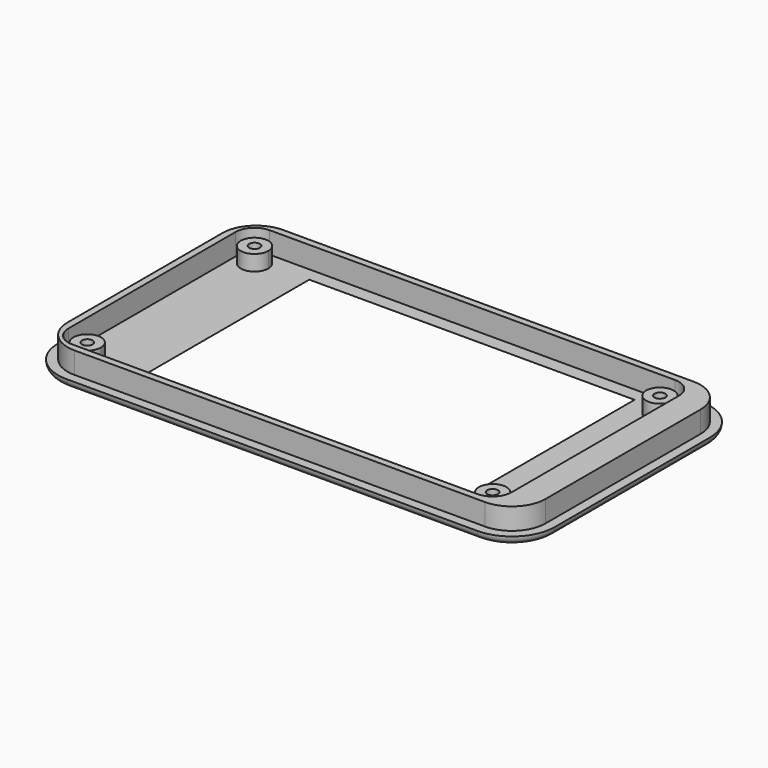
from build123d import *

# Parameters (mm, degrees)
F1_DEPTH = 5.6
F2_DEPTH = 7
F0_W     = 75.5
F0_H     = 51
F3_DEPTH = 2
F4_R     = 1.99999
F5_SIZE2 = 1.99999
F5_SIZE  = 2.99999
F6_R     = 1.25
F7_DEPTH = 5


# Not quite as in the source:
# - a fillet or chamfer is up to 0.001 mm smaller than in the source, because OpenCascade refuses the exact size


with BuildPart() as f1:
    # F0 (on Top) → F1 (new body)
    with BuildSketch(Plane.XY):
        with BuildLine():
            ThreePointArc((-34.4414402544, 28.4581715763), (-31.2414402544, 25.2581715763), (-28.0414402544, 28.4581715763))
            ThreePointArc((-28.0414402544, 28.4581715763), (-28.9786985547, 30.7209132761), (-31.2414402544, 31.6581715763))
            ThreePointArc((-31.2414402544, 31.6581715763), (-33.5041819542, 30.7209132761), (-34.4414402544, 28.4581715763))
        make_face()
    extrude(amount=F1_DEPTH)



with BuildPart() as f1b:
    # F0 (on Top) → F1, piece 2 (new body)
    with BuildSketch(Plane.XY):
        with BuildLine():
            ThreePointArc((-28.0414402544, -20.0818284237), (-31.2414402544, -16.8818284237), (-34.4414402544, -20.0818284237))
            ThreePointArc((-34.4414402544, -20.0818284237), (-33.5041819542, -22.3445701235), (-31.2414402544, -23.2818284237))
            ThreePointArc((-31.2414402544, -23.2818284237), (-28.9786985547, -22.3445701235), (-28.0414402544, -20.0818284237))
        make_face()
    extrude(amount=F1_DEPTH)


with BuildPart() as f1c:
    # F0 (on Top) → F1, piece 3 (new body)
    with BuildSketch(Plane.XY):
        with BuildLine():
            ThreePointArc((62.8585597456, -23.2818284237), (65.1213014453, -22.3445701235), (66.0585597456, -20.0818284237))
            ThreePointArc((66.0585597456, -20.0818284237), (60.5958180458, -17.8190867239), (62.8585597456, -23.2818284237))
        make_face()
    extrude(amount=F1_DEPTH)


with BuildPart() as f1d:
    # F0 (on Top) → F1, piece 4 (new body)
    with BuildSketch(Plane.XY):
        with BuildLine():
            ThreePointArc((66.0585597456, 28.4581715763), (65.1213014453, 30.7209132761), (62.8585597456, 31.6581715763))
            ThreePointArc((62.8585597456, 31.6581715763), (60.5958180458, 26.1954298765), (66.0585597456, 28.4581715763))
        make_face()
    extrude(amount=F1_DEPTH)


with BuildPart() as f2:
    # F0 (on Top) → F2 (new body)
    with BuildSketch(Plane.XY):
        with BuildLine():
            Line((65.8985597456, 34.4581715763), (-29.4414402544, 34.4581715763))
            ThreePointArc((-29.4414402544, 34.4581715763), (-34.9568731477, 32.1736044695), (-37.2414402544, 26.6581715763))
            Line((-37.2414402544, 26.6581715763), (-37.2414402544, -18.2818284237))
            ThreePointArc((-37.2414402544, -18.2818284237), (-34.9568731477, -23.797261317), (-29.4414402544, -26.0818284237))
            Line((-29.4414402544, -26.0818284237), (65.8985597456, -26.0818284237))
            ThreePointArc((65.8985597456, -26.0818284237), (71.4139926388, -23.797261317), (73.6985597456, -18.2818284237))
            Line((73.6985597456, -18.2818284237), (73.6985597456, 26.6581715763))
            ThreePointArc((73.6985597456, 26.6581715763), (71.4139926388, 32.1736044695), (65.8985597456, 34.4581715763))
        make_face()
        with BuildLine():
            ThreePointArc((62.8585597456, 32.8581709981), (65.9698291739, 31.5694410047), (67.2585591674, 28.4581715763))
            Line((67.2585591674, 28.4581715763), (67.2585591674, -20.0818284237))
            ThreePointArc((67.2585591674, -20.0818284237), (65.9698291739, -23.1930978521), (62.8585597456, -24.4818278456))
            Line((62.8585597456, -24.4818278456), (-31.2414402544, -24.4818278456))
            ThreePointArc((-31.2414402544, -24.4818278456), (-34.3527096828, -23.1930978521), (-35.6414396763, -20.0818284237))
            Line((-35.6414396763, -20.0818284237), (-35.6414396763, 28.4581715763))
            ThreePointArc((-35.6414396763, 28.4581715763), (-34.3527096828, 31.5694410047), (-31.2414402544, 32.8581709981))
            Line((-31.2414402544, 32.8581709981), (62.8585597456, 32.8581709981))
        make_face(mode=Mode.SUBTRACT)
    extrude(amount=F2_DEPTH)


with BuildPart() as f1_1:
    add(f1.part)

    add(f1b.part)  # F3 merges F1b

    add(f1c.part)  # F3 merges F1c

    add(f1d.part)  # F3 merges F1d

    add(f2.part)  # F3 merges F2
    # F0 (on Top) → F3 (join)
    with BuildSketch(Plane.XY):
        with BuildLine():
            Line((65.8985597456, 36.6581715763), (-29.4414402544, 36.6581715763))
            ThreePointArc((-29.4414402544, 36.6581715763), (-36.5125080663, 33.7292393881), (-39.4414402544, 26.6581715763))
            Line((-39.4414402544, 26.6581715763), (-39.4414402544, -18.2818284237))
            ThreePointArc((-39.4414402544, -18.2818284237), (-36.5125080663, -25.3528962356), (-29.4414402544, -28.2818284237))
            Line((-29.4414402544, -28.2818284237), (65.8985597456, -28.2818284237))
            ThreePointArc((65.8985597456, -28.2818284237), (72.9696275574, -25.3528962356), (75.8985597456, -18.2818284237))
            Line((75.8985597456, -18.2818284237), (75.8985597456, 26.6581715763))
            ThreePointArc((75.8985597456, 26.6581715763), (72.9696275574, 33.7292393881), (65.8985597456, 36.6581715763))
        make_face()
        with BuildLine():
            ThreePointArc((-37.2414402544, 26.6581715763), (-34.9568731477, 32.1736044695), (-29.4414402544, 34.4581715763))
            Line((-29.4414402544, 34.4581715763), (65.8985597456, 34.4581715763))
            ThreePointArc((65.8985597456, 34.4581715763), (71.4139926388, 32.1736044695), (73.6985597456, 26.6581715763))
            Line((73.6985597456, 26.6581715763), (73.6985597456, -18.2818284237))
            ThreePointArc((73.6985597456, -18.2818284237), (71.4139926388, -23.797261317), (65.8985597456, -26.0818284237))
            Line((65.8985597456, -26.0818284237), (-29.4414402544, -26.0818284237))
            ThreePointArc((-29.4414402544, -26.0818284237), (-34.9568731477, -23.797261317), (-37.2414402544, -18.2818284237))
            Line((-37.2414402544, -18.2818284237), (-37.2414402544, 26.6581715763))
        make_face(mode=Mode.SUBTRACT)
        with BuildLine():
            Line((67.2585591674, -20.0818284237), (67.2585591674, 28.4581715763))
            ThreePointArc((67.2585591674, 28.4581715763), (65.9698291739, 31.5694410047), (62.8585597456, 32.8581709981))
            Line((62.8585597456, 32.8581709981), (-31.2414402544, 32.8581709981))
            ThreePointArc((-31.2414402544, 32.8581709981), (-34.3527096828, 31.5694410047), (-35.6414396763, 28.4581715763))
            Line((-35.6414396763, 28.4581715763), (-35.6414396763, -20.0818284237))
            ThreePointArc((-35.6414396763, -20.0818284237), (-34.3527096828, -23.1930978521), (-31.2414402544, -24.4818278456))
            Line((-31.2414402544, -24.4818278456), (62.8585597456, -24.4818278456))
            ThreePointArc((62.8585597456, -24.4818278456), (65.9698291739, -23.1930978521), (67.2585591674, -20.0818284237))
        make_face()
        with BuildLine():
            ThreePointArc((-34.4414402544, 28.4581715763), (-33.5041819542, 30.7209132761), (-31.2414402544, 31.6581715763))
            Line((-31.2414402544, 31.6581715763), (62.8585597456, 31.6581715763))
            ThreePointArc((62.8585597456, 31.6581715763), (65.1213014453, 30.7209132761), (66.0585597456, 28.4581715763))
            Line((66.0585597456, 28.4581715763), (66.0585597456, -20.0818284237))
            ThreePointArc((66.0585597456, -20.0818284237), (65.1213014453, -22.3445701235), (62.8585597456, -23.2818284237))
            Line((62.8585597456, -23.2818284237), (-31.2414402544, -23.2818284237))
            ThreePointArc((-31.2414402544, -23.2818284237), (-33.5041819542, -22.3445701235), (-34.4414402544, -20.0818284237))
            Line((-34.4414402544, -20.0818284237), (-34.4414402544, 28.4581715763))
        make_face(mode=Mode.SUBTRACT)
        with BuildLine():
            ThreePointArc((-31.2414402544, 31.6581715763), (-28.9786985547, 30.7209132761), (-28.0414402544, 28.4581715763))
            ThreePointArc((-28.0414402544, 28.4581715763), (-31.2414402544, 25.2581715763), (-34.4414402544, 28.4581715763))
            Line((-34.4414402544, 28.4581715763), (-34.4414402544, -20.0818284237))
            ThreePointArc((-34.4414402544, -20.0818284237), (-31.2414402544, -16.8818284237), (-28.0414402544, -20.0818284237))
            ThreePointArc((-28.0414402544, -20.0818284237), (-28.9786985547, -22.3445701235), (-31.2414402544, -23.2818284237))
            Line((-31.2414402544, -23.2818284237), (62.8585597456, -23.2818284237))
            ThreePointArc((62.8585597456, -23.2818284237), (60.5958180458, -17.8190867239), (66.0585597456, -20.0818284237))
            Line((66.0585597456, -20.0818284237), (66.0585597456, 28.4581715763))
            ThreePointArc((66.0585597456, 28.4581715763), (60.5958180458, 26.1954298765), (62.8585597456, 31.6581715763))
            Line((62.8585597456, 31.6581715763), (-31.2414402544, 31.6581715763))
        make_face()
        with Locations((18.2285597456, 4.1881715763)):
            Rectangle(F0_W, F0_H, mode=Mode.SUBTRACT)
    extrude(amount=F3_DEPTH)

    # F4 (radius 2 in the source; OpenCascade refuses exactly that, so slightly less here)
    f4_edges = [f1_1.edges().sort_by_distance(p)[0] for p in [
        (-36.512508, -25.352896, 0),
    ]]
    fillet(f4_edges, radius=F4_R)

    # F5 (size 3 and 2 in the source; OpenCascade refuses exactly that, so slightly less here)
    f5_edges = [f1_1.edges().sort_by_distance(p)[0] for p in [
        (18.22856, 29.688172, 0),
        (-19.52144, 4.188172, 0),
        (18.22856, -21.311828, 0),
        (55.97856, 4.188172, 0),
    ]]
    f5_side = f1_1.faces().sort_by_distance((-34.200797, -23.041185, 0))[0]
    chamfer(f5_edges, length=F5_SIZE, length2=F5_SIZE2, reference=f5_side)

    # F6 (on face) → F7 (cut)
    with BuildSketch(Plane.XY.offset(5.6)):
        with Locations((-31.2414402544, 28.4581715763)):
            Circle(F6_R)
        with Locations((-31.2414402544, -20.0818284237)):
            Circle(F6_R)
        with Locations((62.8585597456, -20.0818284237)):
            Circle(F6_R)
        with Locations((62.8585597456, 28.4581715763)):
            Circle(F6_R)
    extrude(amount=-F7_DEPTH, mode=Mode.SUBTRACT)


solid = f1_1.part
